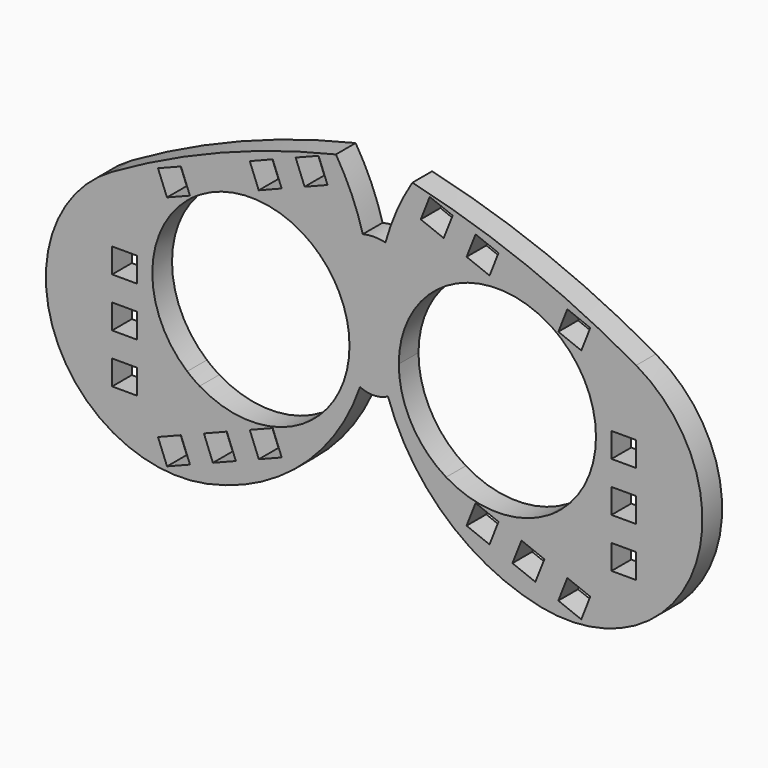
from build123d import *

# Parameters (mm, degrees)
F1_DEPTH = 3
F2_W     = 2.9827502628
F2_H     = 3
F2_W_2   = 2.9913751314
F2_W_3   = 3
F3_DEPTH = 25


# Not quite as in the source:
# - ends of sketch curves that miss each other by under 0.0002 mm in the source are joined


with BuildPart() as f1:
    # F0 (on Front) → F1 (new body)
    with BuildSketch(Plane.XZ):
        with BuildLine():
            ThreePointArc((-65.4990487043, 31.9219294953), (-59.2590567172, 33.6719294953), (-53.01906473, 31.9219294953))
            Line((-53.01906473, 31.9219294953), (-45.1069841329, 31.9219294953))
            ThreePointArc((-45.1069841329, 31.9219294953), (-45.3487223927, 33.0483271736), (-45.635105941, 34.1642095953))
            ThreePointArc((-45.635105941, 34.1642095953), (-47.0071291889, 38.0195574022), (-48.9092989792, 41.6428024387))
            ThreePointArc((-48.9092989792, 41.6428024387), (-62.9189036621, 37.276531414), (-76.1468158191, 30.9239188806))
            ThreePointArc((-76.1468158191, 30.9239188806), (-84.213049611, 16.9468180053), (-76.0504636415, 3.0257667966))
            ThreePointArc((-76.0504636415, 3.0257667966), (-76.029966864, 3.0142304296), (-76.0094479368, 3.0027335048))
            ThreePointArc((-76.0094479368, 3.0027335048), (-70.4614460946, 1.0953454703), (-64.596721114, 1.2484939552))
            ThreePointArc((-64.596721114, 1.2484939552), (-55.9033559949, 4.8590380101), (-49.1550909719, 11.4219294953))
            Line((-49.1550909719, 11.4219294953), (-53.01906473, 11.4219294953))
            ThreePointArc((-53.01906473, 11.4219294953), (-59.2590567172, 9.6719294953), (-65.4990487043, 11.4219294953))
            Line((-65.4990487043, 11.4219294953), (-67.0090567172, 11.4219294953))
            Line((-67.0090567172, 11.4219294953), (-67.0090567172, 12.5101883944))
            ThreePointArc((-67.0090567172, 12.5101883944), (-71.2590567172, 21.6719294953), (-67.0090567172, 30.8336705962))
            Line((-67.0090567172, 30.8336705962), (-67.0090567172, 31.9219294953))
            Line((-67.0090567172, 31.9219294953), (-65.4990487043, 31.9219294953))
        make_face()
        with BuildLine():
            ThreePointArc((-42.8830074933, 34.1642095953), (-43.1693910416, 33.0483271736), (-43.4111293014, 31.9219294953))
            Line((-43.4111293014, 31.9219294953), (-35.4990487043, 31.9219294953))
            ThreePointArc((-35.4990487043, 31.9219294953), (-29.2590567172, 33.6719294953), (-23.01906473, 31.9219294953))
            Line((-23.01906473, 31.9219294953), (-21.5090567172, 31.9219294953))
            Line((-21.5090567172, 31.9219294953), (-21.5090567172, 30.8336705962))
            ThreePointArc((-21.5090567172, 30.8336705962), (-18.3732861886, 26.7216819645), (-17.2590567172, 21.6719294953))
            ThreePointArc((-17.2590567172, 21.6719294953), (-18.3732861886, 16.6221770261), (-21.5090567172, 12.5101883944))
            Line((-21.5090567172, 12.5101883944), (-21.5090567172, 11.4219294953))
            Line((-21.5090567172, 11.4219294953), (-23.01906473, 11.4219294953))
            ThreePointArc((-23.01906473, 11.4219294953), (-29.2590567172, 9.6719294953), (-35.4990487043, 11.4219294953))
            Line((-35.4990487043, 11.4219294953), (-39.3630224624, 11.4219294953))
            ThreePointArc((-39.3630224624, 11.4219294953), (-32.6147574394, 4.8590380101), (-23.9213923203, 1.2484939552))
            ThreePointArc((-23.9213923203, 1.2484939552), (-18.0566673397, 1.0953454703), (-12.5086654975, 3.0027335048))
            ThreePointArc((-12.5086654975, 3.0027335048), (-12.4881465704, 3.0142304296), (-12.4676497928, 3.0257667966))
            ThreePointArc((-12.4676497928, 3.0257667966), (-4.3050638233, 16.9468180053), (-12.3712976152, 30.9239188806))
            ThreePointArc((-12.3712976152, 30.9239188806), (-25.5992097722, 37.276531414), (-39.6088144552, 41.6428024387))
            ThreePointArc((-39.6088144552, 41.6428024387), (-41.5109842454, 38.0195574022), (-42.8830074933, 34.1642095953))
        make_face()
        with BuildLine():
            Line((-43.5487545967, 21.6719294953), (-44.9693588376, 21.6719294953))
            ThreePointArc((-44.9693588376, 21.6719294953), (-45.3908188129, 19.6558686516), (-45.9763922185, 17.6812209304))
            ThreePointArc((-45.9763922185, 17.6812209304), (-44.2636810752, 17.3202159397), (-42.5729841678, 17.7732590184))
            ThreePointArc((-42.5729841678, 17.7732590184), (-43.1391404553, 19.7030043482), (-43.5487545967, 21.6719294953))
        make_face()
        with BuildLine():
            ThreePointArc((-43.559121813, 21.7346880473), (-43.5539581146, 21.7033054824), (-43.5487545967, 21.6719294953))
            Line((-43.5487545967, 21.6719294953), (-41.2590567172, 21.6719294953))
            ThreePointArc((-41.2590567172, 21.6719294953), (-39.7204118838, 27.550708967), (-35.4990487043, 31.9219294953))
            Line((-35.4990487043, 31.9219294953), (-43.4111293014, 31.9219294953))
            ThreePointArc((-43.4111293014, 31.9219294953), (-43.9370167563, 26.8348735037), (-43.559121813, 21.7346880473))
        make_face()
        with BuildLine():
            ThreePointArc((-53.01906473, 31.9219294953), (-48.7977015505, 27.550708967), (-47.2590567172, 21.6719294953))
            Line((-47.2590567172, 21.6719294953), (-44.9693588376, 21.6719294953))
            ThreePointArc((-44.9693588376, 21.6719294953), (-44.9641553197, 21.7033054824), (-44.9589916213, 21.7346880473))
            ThreePointArc((-44.9589916213, 21.7346880473), (-44.581096678, 26.8348735037), (-45.1069841329, 31.9219294953))
            Line((-45.1069841329, 31.9219294953), (-53.01906473, 31.9219294953))
        make_face()
        with BuildLine():
            Line((-44.9693588376, 21.6719294953), (-47.2590567172, 21.6719294953))
            ThreePointArc((-47.2590567172, 21.6719294953), (-48.7977015505, 15.7931500236), (-53.01906473, 11.4219294953))
            Line((-53.01906473, 11.4219294953), (-49.1550909719, 11.4219294953))
            ThreePointArc((-49.1550909719, 11.4219294953), (-47.3455028522, 14.4397298666), (-45.9763922185, 17.6812209304))
            ThreePointArc((-45.9763922185, 17.6812209304), (-45.3908188129, 19.6558686516), (-44.9693588376, 21.6719294953))
        make_face()
        with BuildLine():
            Line((-41.2590567172, 21.6719294953), (-43.5487545967, 21.6719294953))
            ThreePointArc((-43.5487545967, 21.6719294953), (-43.1391404553, 19.7030043482), (-42.5729841678, 17.7732590184))
            ThreePointArc((-42.5729841678, 17.7732590184), (-41.1945750254, 14.4830849229), (-39.3630224624, 11.4219294953))
            Line((-39.3630224624, 11.4219294953), (-35.4990487043, 11.4219294953))
            ThreePointArc((-35.4990487043, 11.4219294953), (-39.7204118838, 15.7931500236), (-41.2590567172, 21.6719294953))
        make_face()
        with BuildLine():
            ThreePointArc((-44.9589916213, 21.7346880473), (-44.9641553197, 21.7033054824), (-44.9693588376, 21.6719294953))
            Line((-44.9693588376, 21.6719294953), (-43.5487545967, 21.6719294953))
            ThreePointArc((-43.5487545967, 21.6719294953), (-43.5539581146, 21.7033054824), (-43.559121813, 21.7346880473))
            ThreePointArc((-43.559121813, 21.7346880473), (-43.9370167563, 26.8348735037), (-43.4111293014, 31.9219294953))
            Line((-43.4111293014, 31.9219294953), (-45.1069841329, 31.9219294953))
            ThreePointArc((-45.1069841329, 31.9219294953), (-44.581096678, 26.8348735037), (-44.9589916213, 21.7346880473))
        make_face()
        with BuildLine():
            ThreePointArc((-45.635105941, 34.1642095953), (-45.3487223927, 33.0483271736), (-45.1069841329, 31.9219294953))
            Line((-45.1069841329, 31.9219294953), (-43.4111293014, 31.9219294953))
            ThreePointArc((-43.4111293014, 31.9219294953), (-43.1693910416, 33.0483271736), (-42.8830074933, 34.1642095953))
            ThreePointArc((-42.8830074933, 34.1642095953), (-44.2590567172, 34.327758758), (-45.635105941, 34.1642095953))
        make_face()
        with BuildLine():
            Line((-67.0090567172, 11.4219294953), (-65.4990487043, 11.4219294953))
            ThreePointArc((-65.4990487043, 11.4219294953), (-66.2751842679, 11.9367379619), (-67.0090567172, 12.5101883944))
            Line((-67.0090567172, 12.5101883944), (-67.0090567172, 11.4219294953))
        make_face()
        with BuildLine():
            ThreePointArc((-21.5090567172, 12.5101883944), (-22.2429291664, 11.9367379619), (-23.01906473, 11.4219294953))
            Line((-23.01906473, 11.4219294953), (-21.5090567172, 11.4219294953))
            Line((-21.5090567172, 11.4219294953), (-21.5090567172, 12.5101883944))
        make_face()
        with BuildLine():
            Line((-21.5090567172, 31.9219294953), (-23.01906473, 31.9219294953))
            ThreePointArc((-23.01906473, 31.9219294953), (-22.2429291664, 31.4071210287), (-21.5090567172, 30.8336705962))
            Line((-21.5090567172, 30.8336705962), (-21.5090567172, 31.9219294953))
        make_face()
        with BuildLine():
            ThreePointArc((-67.0090567172, 30.8336705962), (-66.2751842679, 31.4071210287), (-65.4990487043, 31.9219294953))
            Line((-65.4990487043, 31.9219294953), (-67.0090567172, 31.9219294953))
            Line((-67.0090567172, 31.9219294953), (-67.0090567172, 30.8336705962))
        make_face()
    extrude(amount=F1_DEPTH)

    # F2 (on face) → F3 (cut)
    with BuildSketch(Plane.XZ.offset(3)):
        Polygon((-67.7719824437, 5.4260265126), (-70.5635935688, 4.3274331729), (-69.4650002292, 1.5358220478), (-66.673389104, 2.6344153875), align=None)
        Polygon((-29.1209643657, 8.7218065315), (-31.9125754908, 9.8203998712), (-33.0111329333, 7.0288799637), (-30.2195218081, 5.930286624), align=None)
        Polygon((-23.5377421156, 6.5246198522), (-26.3293532407, 7.6232131919), (-27.4279286318, 4.8316476756), (-24.6363175066, 3.7330543359), align=None)
        Polygon((-19.0531132051, 1.5358220478), (-17.9545198655, 4.3274331729), (-20.7461309906, 5.4260265126), (-21.8447243303, 2.6344153875), align=None)
        with Locations((-13.8799224838, 9.4239312787)):
            Rectangle(F2_W, F2_H)
        with Locations((-13.8756100495, 15.4239250796)):
            Rectangle(F2_W_2, F2_H)
        with Locations((-13.8712976152, 21.4239188806)):
            Rectangle(F2_W_3, F2_H)
        Polygon((-19.0457892079, 30.3481052815), (-17.9545198238, 33.1211056658), (-20.7461309906, 34.2196988996), (-21.837400333, 31.4466986212), align=None)
        Polygon((-29.120964366, 37.5154789187), (-31.9125754912, 38.6140722584), (-33.0038447503, 35.8410721917), (-30.2122336251, 34.742478852), align=None)
        Polygon((-34.7041866163, 39.712665598), (-37.4957977415, 40.8112589377), (-38.5870669589, 38.0382589769), (-35.7954558337, 36.9396656372), align=None)
        Polygon((-67.7719824437, 34.2196988996), (-70.5635935688, 33.12110556), (-69.4723242264, 30.3481052815), (-66.6807131013, 31.4466986212), align=None)
        Polygon((-55.5142686841, 35.8410721917), (-56.6055380681, 38.614072576), (-59.3971490683, 37.5154789187), (-58.3058798092, 34.742478852), align=None)
        Polygon((-49.9310464754, 38.0382589769), (-51.0223158595, 40.8112593612), (-53.813926818, 39.712665598), (-52.7226576006, 36.9396656372), align=None)
        with Locations((-74.6468158191, 21.4239188806)):
            Rectangle(F2_W_3, F2_H)
        with Locations((-74.6468158191, 9.4239419771)):
            Rectangle(F2_W_3, F2_H)
        Polygon((-61.0901668537, 4.8316020668), (-62.1887601934, 7.623213192), (-64.9803713186, 6.5246198523), (-63.8817779789, 3.7330087272), align=None)
        Polygon((-55.5069446035, 7.0287887462), (-56.6055379431, 9.8203998713), (-59.3971490683, 8.7218065317), (-58.2985557286, 5.9301954065), align=None)
        with Locations((-74.6468158191, 15.4239304289)):
            Rectangle(F2_W_3, F2_H)
    extrude(amount=-F3_DEPTH, mode=Mode.SUBTRACT)


solid = f1.part
